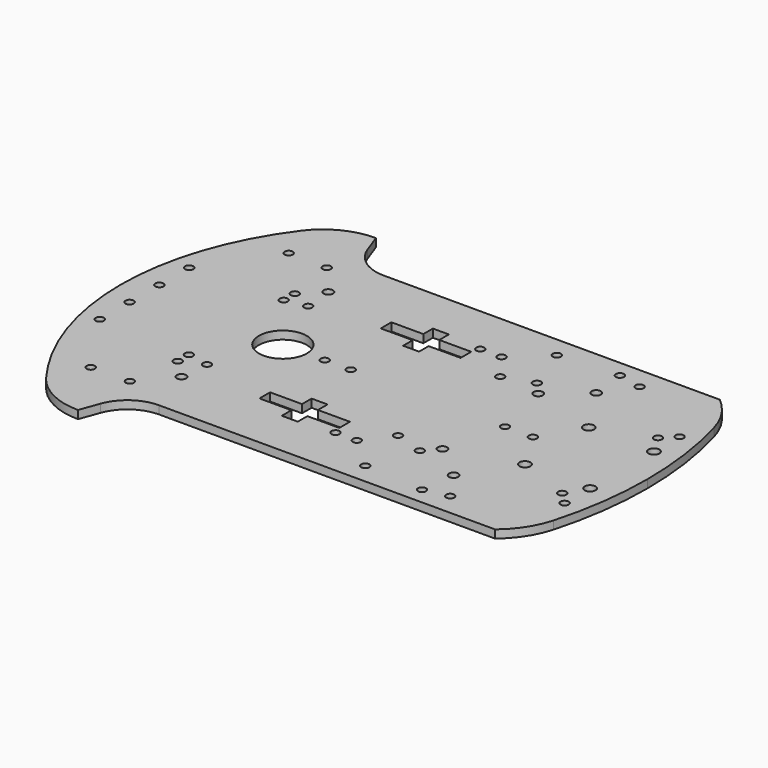
from build123d import *

# Parameters (mm, degrees)
F1_DEPTH = 1.525
F2_R     = 9
F2_R_2   = 1.535
F2_R_3   = 1.75
F2_R_4   = 2.035
F3_DEPTH = 3.051
F6_DEPTH = 3.05


# Not quite as in the source:
# - a pattern or mirror of a feature is missing from the dataset's text; its kind, count and spacing are read off the source's solid


with BuildPart() as f1:
    # F0 (on Top) → F1 (new body, symmetric)
    with BuildSketch(Plane.XY):
        with BuildLine():
            Line((122, 52.8), (-4.2365988975, 52.8))
            ThreePointArc((-4.2365988975, 52.8), (-12.8402454427, 55.5127193357), (-18.3319882093, 62.6696978501))
            Line((-18.3319882093, 62.6696978501), (-21, 70))
            ThreePointArc((-21, 70), (-32.1803398875, 67.360679775), (-41, 60))
            ThreePointArc((-41, 60), (-55.8683298051, 31.6227766017), (-61, 0))
            Line((-61, 0), (137, 0))
            ThreePointArc((137, 0), (135.6994290201, 19.038602614), (131.8218801501, 37.7234758844))
            ThreePointArc((131.8218801501, 37.7234758844), (128.067905641, 46.0154645332), (122, 52.8))
        make_face()
    extrude(amount=F1_DEPTH, both=True)

    # F2 (on face) → F3 (cut, through all)
    with BuildSketch(Plane.XY.offset(1.525)):
        Circle(F2_R)
        with Locations((-52, 21)):
            Circle(F2_R_2)
        with Locations((-52, 7)):
            Circle(F2_R_2)
        with Locations((-35, 46.5)):
            Circle(F2_R_2)
        with Locations((-20.5, 46.25)):
            Circle(F2_R_2)
        with Locations((-17.5, 27.5)):
            Circle(F2_R_2)
        with Locations((-17.5, 22.25)):
            Circle(F2_R_2)
        with Locations((-10.5, 34.5)):
            Circle(F2_R_3)
        with Locations((-9.5, 23.75)):
            Circle(F2_R_2)
        with Locations((15.75, 0)):
            Circle(F2_R_2)
        with Locations((25.5, 0)):
            Circle(F2_R_2)
        with Locations((47, 34)):
            Circle(F2_R_2)
        with Locations((55, 34)):
            Circle(F2_R_2)
        with Locations((62.5, 24)):
            Circle(F2_R_2)
        with Locations((67, 45)):
            Circle(F2_R_2)
        with Locations((73.5, 27.5)):
            Circle(F2_R_2)
        with Locations((78, 22.5)):
            Circle(F2_R_3)
        with Locations((83.5, 0)):
            Circle(F2_R_2)
        with Locations((94, 0)):
            Circle(F2_R_2)
        with Locations((91, 33.5)):
            Circle(F2_R_3)
        with Locations((89.5, 46.5)):
            Circle(F2_R_2)
        with Locations((98.5, 44.5)):
            Circle(F2_R_2)
        with Locations((103, 15)):
            Circle(F2_R_4)
        with Locations((123, 22.5)):
            Circle(F2_R_2)
        with Locations((127.5, 27)):
            Circle(F2_R_2)
        with Locations((127.5, 15)):
            Circle(F2_R_4)
    extrude(amount=-F3_DEPTH, mode=Mode.SUBTRACT)

    # F4: F1 across face


with BuildPart() as f1_1:
    add(f1.part)
    add(f1.part.mirror(Plane(origin=(54.5, 0, 0), x_dir=(1, 0, 0), z_dir=(0, -1, 0))))

    # F5 (on face) → F6 (cut, through all)
    with BuildSketch(Plane.XY.offset(1.525)):
        Polygon((46, 31), (34, 31), (34, 35.5), (28, 35.5), (28, 31), (16, 31), (16, 26), (28, 26), (28, 21.5), (34, 21.5), (34, 26), (46, 26), align=None)
    f6 = extrude(amount=-F6_DEPTH, mode=Mode.SUBTRACT)

    # F6_copies: F6 across plane
    add(f6.mirror(Plane(origin=(0, 0, 0), x_dir=(0, 0, -1), z_dir=(0, -1, 0))), mode=Mode.SUBTRACT)


solid = f1_1.part
